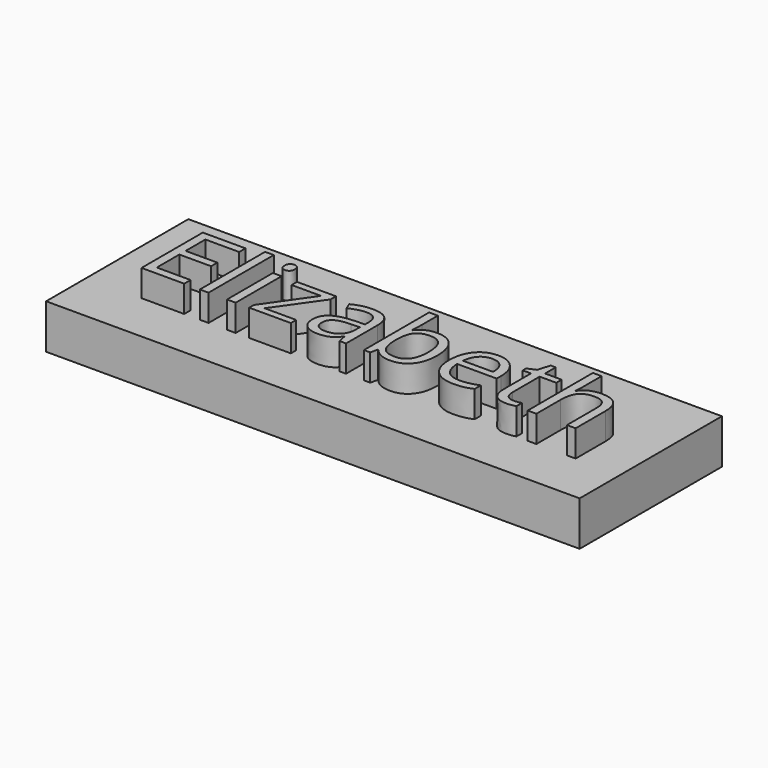
from build123d import *

# Parameters (mm, degrees)
F0_W         = 60
F0_H         = 20
F1_DEPTH     = 5
F2_TEXT_SIZE = 12.0595439985
F3_DEPTH     = 3


# Not quite as in the source:
# - Text() gives the source's letters only with a copy of the font that has no kerning and outlines rounded to 1/6400 em; it was checked with that copy


with BuildPart() as f1:
    # F0 (on Top) → F1 (new body)
    with BuildSketch(Plane.XY):
        Rectangle(F0_W, F0_H)
    extrude(amount=F1_DEPTH)

    # F2 (on face) → F3 (join)
    with BuildSketch(Plane.XY.offset(5)):
        with Locations((-25, -4.3110626099)):
            Text('Elizabeth', F2_TEXT_SIZE, font='Open Sans', text_align=(TextAlign.LEFT, TextAlign.BOTTOM))
    extrude(amount=F3_DEPTH)


solid = f1.part
